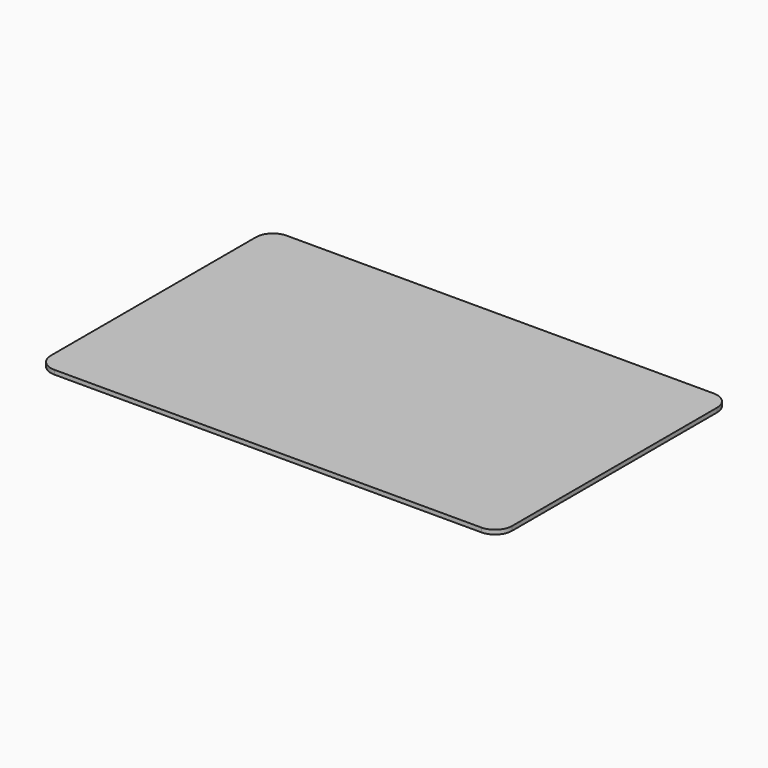
from build123d import *

# Parameters (mm, degrees)
F1_DEPTH = 0.79375


# Not quite as in the source:
# - a length typed as a fraction of an inch, garbled in the dataset ("3 / 203.2 mm" for 3/8 in), is restored


with BuildPart() as f1:
    # F0 (on Top) → F1 (new body)
    with BuildSketch(Plane.XY):
        with BuildLine():
            ThreePointArc((42.8625, 23.8125), (41.9325640303, 26.0575640303), (39.6875, 26.9875))
            Line((39.6875, 26.9875), (-39.6875, 26.9875))
            ThreePointArc((-39.6875, 26.9875), (-41.9325640303, 26.0575640303), (-42.8625, 23.8125))
            Line((-42.8625, 23.8125), (-42.8625, -23.8125))
            ThreePointArc((-42.8625, -23.8125), (-41.9325640303, -26.0575640303), (-39.6875, -26.9875))
            Line((-39.6875, -26.9875), (39.6875, -26.9875))
            ThreePointArc((39.6875, -26.9875), (41.9325640303, -26.0575640303), (42.8625, -23.8125))
            Line((42.8625, -23.8125), (42.8625, 23.8125))
        make_face()
    extrude(amount=F1_DEPTH)


solid = f1.part
